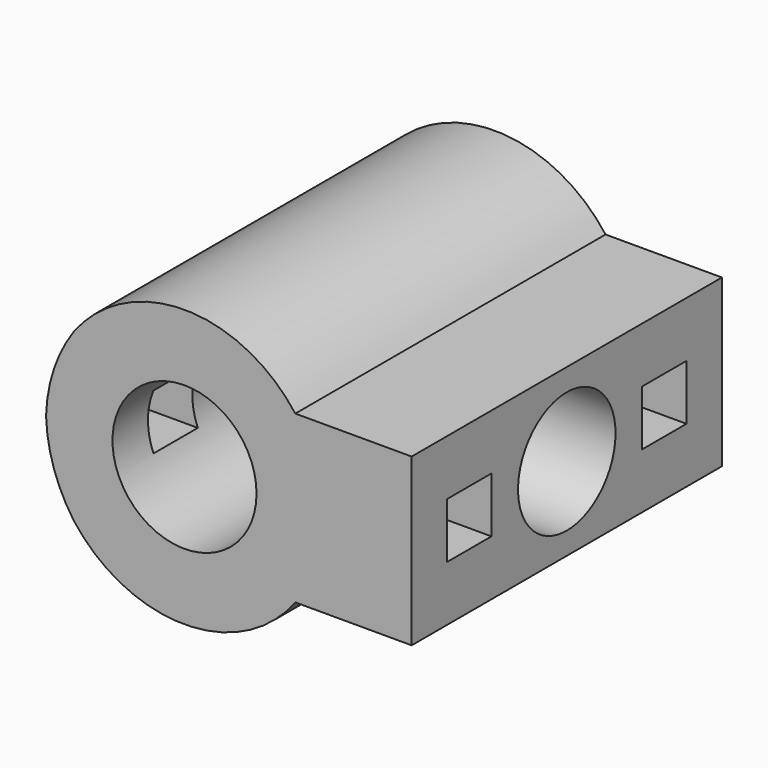
from build123d import *

# Parameters (mm, degrees)
F0_W        = 70
F0_H        = 30
F1_DEPTH    = 66
F3_DEPTH    = 70
F4_R        = 13
F5_DEPTH    = 71
F6_W        = 10
F6_H        = 10
F6_R        = 11
F7_DEPTH    = 70
F8_T1_DEPTH = 149.09177361
F9_T1_DEPTH = 8.9088895058
F9_T3_DEPTH = 6.9088895058


# Not quite as in the source:
# - a fillet or chamfer that OpenCascade refuses, or shapes differently, is made with other operations: its cross-section is extruded or revolved along the edge and cut away or added


with BuildPart() as f1:
    # F0 (on Right) → F1 (new body)
    with BuildSketch(Plane.YZ):
        Rectangle(F0_W, F0_H)
    extrude(amount=-F1_DEPTH)

    # F2 (on face) → F3 (join)
    with BuildSketch(Plane.XZ.offset(35)):
        with BuildLine():
            Line((-41, 15), (-21, 15))
            ThreePointArc((-21, 15), (-41, 25), (-61, 15))
            Line((-61, 15), (-41, 15))
        make_face()
        with BuildLine():
            ThreePointArc((-61, -15), (-41, -25), (-21, -15))
            Line((-21, -15), (-61, -15))
        make_face()
    extrude(amount=-F3_DEPTH)

    # F4 (on face) → F5 (cut)
    with BuildSketch(Plane.XZ.offset(35)):
        with Locations((-41, 0)):
            Circle(F4_R)
    extrude(amount=-F5_DEPTH, mode=Mode.SUBTRACT)

    # F6 (on face) → F7 (cut)
    with BuildSketch(Plane.YZ):
        with Locations((-22, 0)):
            Rectangle(F6_W, F6_H)
        Circle(F6_R)
        with Locations((22, 0)):
            Rectangle(F6_W, F6_H)
    extrude(amount=-F7_DEPTH, mode=Mode.SUBTRACT)

    # F8: fillet of radius 27.5220346111 on 2 edges, made by hand

    # F8_s2 → F8_t1 (cut)
    with BuildSketch(Plane.XZ.offset(-74.545886805)):
        with BuildLine():
            ThreePointArc((-66, -0.818354722), (-64.7202462083, 7.4765284314), (-61, 15))
            Line((-61, 15), (-66, 15))
            Line((-66, 15), (-66, -0.818354722))
        make_face()
        with BuildLine():
            ThreePointArc((-61, -15), (-64.7202462083, -7.4765284314), (-66, 0.818354722))
            Line((-66, 0.818354722), (-66, -15))
            Line((-66, -15), (-61, -15))
        make_face()
    extrude(amount=F8_T1_DEPTH, mode=Mode.SUBTRACT)

    # F9: fillet of radius 5 on 2 edges, made by hand

    # F9_s2 → F9_t1 (cut)
    with BuildSketch(Plane.XZ.offset(26.5455552471)):
        with BuildLine():
            ThreePointArc((-65.9818255238, 0.1816786841), (-65.9851273284, 0), (-65.9818255238, -0.1816786841))
            ThreePointArc((-65.9818255238, -0.1816786841), (-65.9849780634, -0.0908442999), (-65.9878306136, 0))
            ThreePointArc((-65.9878306136, 0), (-65.9849780634, 0.0908442999), (-65.9818255238, 0.1816786841))
        make_face()
    extrude(amount=F9_T1_DEPTH, mode=Mode.SUBTRACT)

    # F9_s4 → F9_t3 (cut)
    with BuildSketch(Plane.XZ.offset(10.5455552471)):
        with BuildLine():
            ThreePointArc((-65.9818255238, 0.1816786841), (-65.9851273284, 0), (-65.9818255238, -0.1816786841))
            ThreePointArc((-65.9818255238, -0.1816786841), (-65.9849780634, -0.0908442999), (-65.9878306136, 0))
            ThreePointArc((-65.9878306136, 0), (-65.9849780634, 0.0908442999), (-65.9818255238, 0.1816786841))
        make_face()
    extrude(amount=F9_T3_DEPTH, mode=Mode.SUBTRACT)


solid = f1.part
